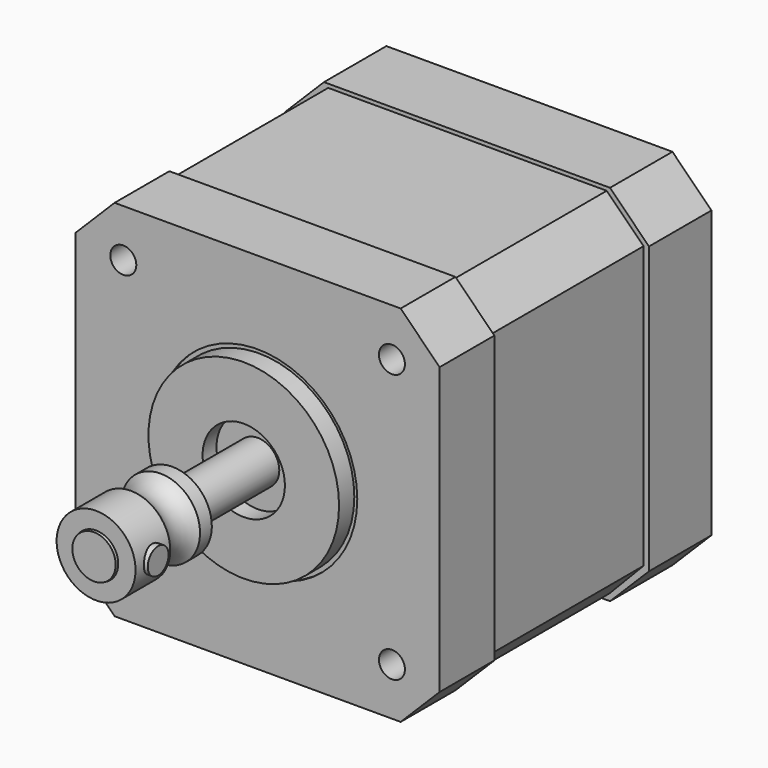
from build123d import *

# Parameters (mm, degrees)
F0_R           = 1.5
F0_R_2         = 11.5
F1_DEPTH       = 7.9
F0_R_3         = 11
F0_R_4         = 4.75
F2_DEPTH       = 9.9
F0_R_5         = 2.5
F3_DEPTH       = 7.9
F4_DEPTH       = 31.5
F5_DEPTH       = 7.7
F7_DEPTH       = 22.3
F8_R           = 1.5
F8_R_2         = 4.75
F9_DEPTH       = 9
F12_R          = 1.5
F13_DEPTH      = 5
F13_DEPTH_BACK = 2


# Not quite as in the source:
# - a feature names something its author has since deleted; it is built from what else it names


with BuildPart() as f1:
    # F0 (on Front) → F1 (new body)
    with BuildSketch(Plane.XZ):
        Polygon((16.5056034888, 21), (-16.5056034888, 21), (-21, 16.5), (-21, -16.5), (-16.5056034888, -21), (16.5056034888, -21), (21, -16.5), (21, 16.5), align=None)
        with Locations((-15.5, -15.5)):
            Circle(F0_R, mode=Mode.SUBTRACT)
        with Locations((15.5, -15.5)):
            Circle(F0_R, mode=Mode.SUBTRACT)
        with Locations((-15.5, 15.5)):
            Circle(F0_R, mode=Mode.SUBTRACT)
        Circle(F0_R_2, mode=Mode.SUBTRACT)
        with Locations((15.5, 15.5)):
            Circle(F0_R, mode=Mode.SUBTRACT)
    extrude(amount=F1_DEPTH)


with BuildPart() as f2:
    # F0 (on Front) → F2 (new body)
    with BuildSketch(Plane.XZ):
        Circle(F0_R_3)
        Circle(F0_R_4, mode=Mode.SUBTRACT)
    extrude(amount=F2_DEPTH)


with BuildPart() as f3:
    # F0 (on Front) → F3 (new body)
    with BuildSketch(Plane.XZ):
        Circle(F0_R_4)
        Circle(F0_R_5, mode=Mode.SUBTRACT)
    extrude(amount=F3_DEPTH)


with BuildPart() as f4:
    # F0 (on Front) → F4 (new body)
    with BuildSketch(Plane.XZ):
        Circle(F0_R_5)
    extrude(amount=F4_DEPTH)


with BuildPart() as f5:
    # F0 (on Front) → F5 (new body)
    with BuildSketch(Plane.XZ):
        Circle(F0_R_2)
        Circle(F0_R_3, mode=Mode.SUBTRACT)
    extrude(amount=F5_DEPTH)


with BuildPart() as f7:
    # F6 (on Front) → F7 (new body)
    with BuildSketch(Plane.XZ):
        Polygon((20.3847829252, 16.3202174008), (16.1285176873, 20.5577779561), (-16.0153234008, 20.5577779561), (-20.5161720514, 16.3202174008), (-20.5161720514, -16.15027152), (-16.3212027401, -20.2703308314), (16.4145436138, -20.2703308314), (20.3847829252, -16.15027152), align=None)
    extrude(amount=-F7_DEPTH)


with BuildPart() as f9:
    # F8 (on face) → F9 (new body)
    with BuildSketch(Plane(origin=(0, 22.3, 0), x_dir=(-1, 0, 0), z_dir=(0, 1, 0))):
        Polygon((16.5031898472, 20.9870020965), (-16.5080171304, 20.9870020965), (-21.0024136416, 16.4870020965), (-21.0024136416, -16.5129979035), (-16.5080171304, -21.0129979035), (16.5031898472, -21.0129979035), (20.9975863584, -16.5129979035), (20.9975863584, 16.4870020965), align=None)
        with Locations((-15.5024136416, -15.5129979035)):
            Circle(F8_R, mode=Mode.SUBTRACT)
        with Locations((15.4975863584, -15.5129979035)):
            Circle(F8_R, mode=Mode.SUBTRACT)
        with Locations((-0.0024136416, -0.0129979035)):
            Circle(F8_R_2, mode=Mode.SUBTRACT)
        with Locations((-15.5024136416, 15.4870020965)):
            Circle(F8_R, mode=Mode.SUBTRACT)
        with Locations((15.4975863584, 15.4870020965)):
            Circle(F8_R, mode=Mode.SUBTRACT)
    extrude(amount=F9_DEPTH)


with BuildPart() as f11:
    # F10 (on Right) → F11 (revolve)
    with BuildSketch(Plane.YZ):
        with BuildLine():
            Line((-31.2, 4.5569573045), (-31.2, 2.5569573045))
            Line((-31.2, 2.5569573045), (-20.2, 2.5569573045))
            Line((-20.2, 2.5569573045), (-20.2, 4.5569573045))
            Line((-20.2, 4.5569573045), (-21.9, 4.5569573045))
            ThreePointArc((-21.9, 4.5569573045), (-24.05, 3.4833402932), (-26.2, 4.5569573045))
            Line((-26.2, 4.5569573045), (-31.2, 4.5569573045))
        make_face()
    revolve(axis=Axis((0, -21.6135401279, 0), (0, -1, 0)))


with BuildPart() as f13:
    # F12 (on Right) → F13 (new body, two sides)
    with BuildSketch(Plane.YZ) as f13_sk:
        with Locations((-28.5, 0)):
            Circle(F12_R)
    extrude(amount=F13_DEPTH)
    extrude(f13_sk.sketch, amount=-F13_DEPTH_BACK)


solid = Compound([f1.part, f2.part, f3.part, f4.part, f5.part, f7.part, f9.part, f11.part, f13.part])
